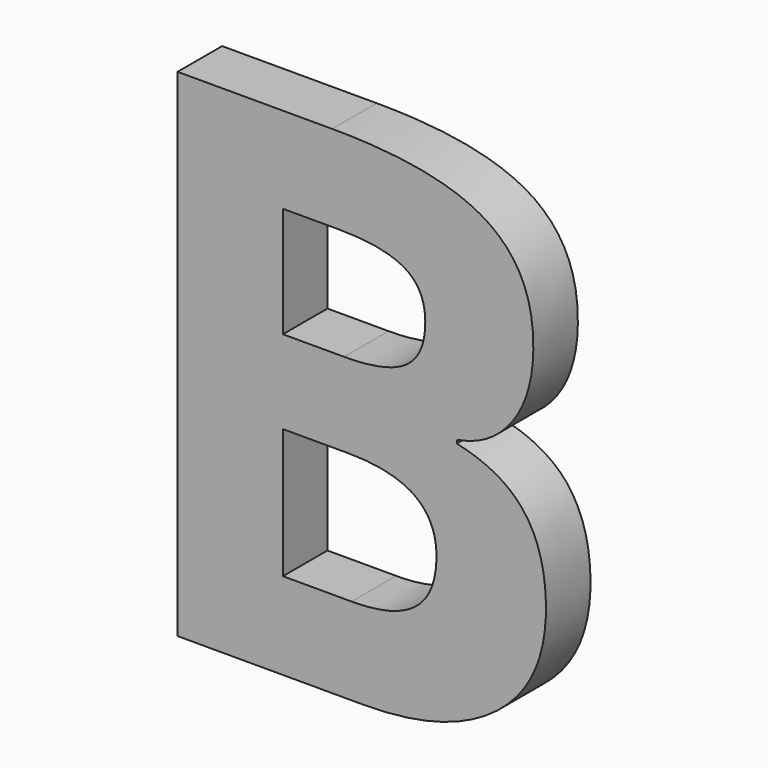
from build123d import *

# Parameters (mm, degrees)
F0_TEXT_SIZE = 62.5
F1_DEPTH     = 5


# Not quite as in the source:
# - Text() gives the source's letters only with a copy of the font that has no kerning and outlines rounded to 1/6400 em; it was checked with that copy


with BuildPart() as f1:
    # F0 (on Front) → F1 (new body)
    with BuildSketch(Plane.XZ):
        with Locations((12.0443906635, -55.2005824447)):
            Text('B', F0_TEXT_SIZE, font='Open Sans', font_style=FontStyle.BOLD, text_align=(TextAlign.LEFT, TextAlign.BOTTOM))
    extrude(amount=F1_DEPTH)


solid = f1.part
